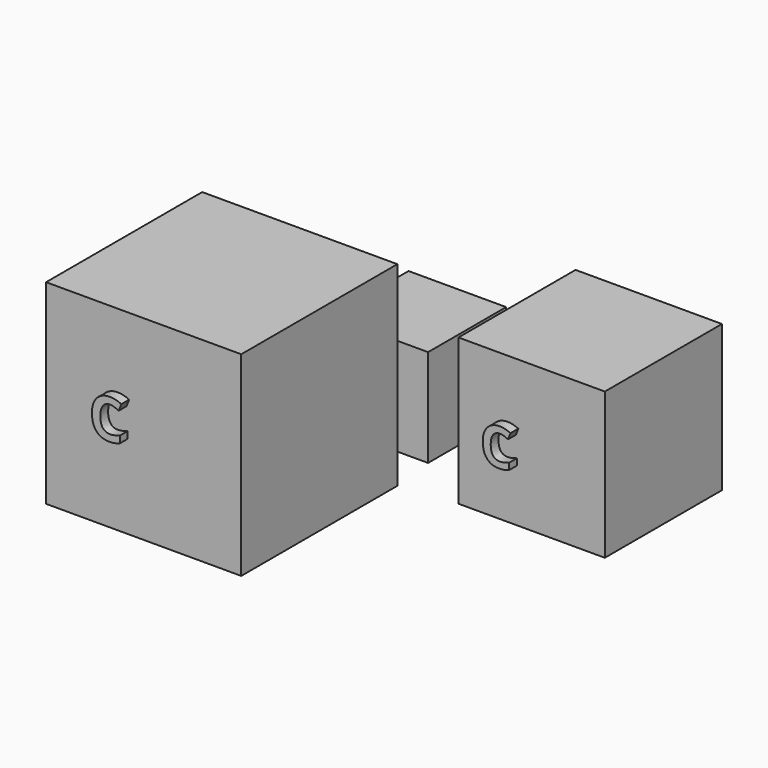
from build123d import *

# Parameters (mm, degrees)
F0_W          = 10
F0_H          = 10
F1_DEPTH      = 10
F2_W          = 20
F2_H          = 20
F3_DEPTH      = 20
F4_W          = 30
F4_H          = 30
F5_DEPTH      = 30
F6_W          = 40
F6_H          = 40
F7_DEPTH      = 40
F8_TEXT_SIZE  = 6.7214882519
F9_DEPTH      = 2
F10_TEXT_SIZE = 10.9602942959
F11_DEPTH     = 2
F12_TEXT_SIZE = 10.4468225295
F13_DEPTH     = 2
F14_TEXT_SIZE = 11.0898968867
F15_DEPTH     = 2


# Not quite as in the source:
# - Text() gives the source's letters only with a copy of the font that has no kerning and outlines rounded to 1/6400 em; it was checked with that copy


with BuildPart() as f1:
    # F0 (on Top) → F1 (new body)
    with BuildSketch(Plane.XY):
        with Locations((-36.1872883514, 28.5152663162)):
            Rectangle(F0_W, F0_H)
    extrude(amount=F1_DEPTH)

    # F8 (on face) → F9 (join)
    with BuildSketch(Plane.XZ.offset(-23.5152663162)):
        with Locations((-40.5598458803, 2.311369055)):
            Text('C', F8_TEXT_SIZE, font='Open Sans', font_style=FontStyle.BOLD, text_align=(TextAlign.LEFT, TextAlign.BOTTOM))
    extrude(amount=F9_DEPTH)


with BuildPart() as f3:
    # F2 (on Top) → F3 (new body)
    with BuildSketch(Plane.XY):
        with Locations((-12.1222923044, 26.0768511578)):
            Rectangle(F2_W, F2_H)
    extrude(amount=F3_DEPTH)

    # F10 (on face) → F11 (join)
    with BuildSketch(Plane.XZ.offset(-16.0768511578)):
        with Locations((-20.2645960653, 5.6796572171)):
            Text('C', F10_TEXT_SIZE, font='Open Sans', font_style=FontStyle.BOLD, text_align=(TextAlign.LEFT, TextAlign.BOTTOM))
    extrude(amount=F11_DEPTH)


with BuildPart() as f5:
    # F4 (on Top) → F5 (new body)
    with BuildSketch(Plane.XY):
        with Locations((25.5017098971, 23.0814629754)):
            Rectangle(F4_W, F4_H)
    extrude(amount=F5_DEPTH)

    # F12 (on face) → F13 (join)
    with BuildSketch(Plane.XZ.offset(-8.0814629754)):
        with Locations((16.4766777307, 10.4974610731)):
            Text('C', F12_TEXT_SIZE, font='Open Sans', font_style=FontStyle.BOLD, text_align=(TextAlign.LEFT, TextAlign.BOTTOM))
    extrude(amount=F13_DEPTH)


with BuildPart() as f7:
    # F6 (on Top) → F7 (new body)
    with BuildSketch(Plane.XY):
        with Locations((-21.0119727999, -13.1803357676)):
            Rectangle(F6_W, F6_H)
    extrude(amount=F7_DEPTH)

    # F14 (on face) → F15 (join)
    with BuildSketch(Plane.XZ.offset(33.1803357676)):
        with Locations((-30.6629557163, 16.8667975813)):
            Text('C', F14_TEXT_SIZE, font='Open Sans', font_style=FontStyle.BOLD, text_align=(TextAlign.LEFT, TextAlign.BOTTOM))
    extrude(amount=F15_DEPTH)


solid = Compound([f1.part, f3.part, f5.part, f7.part])
